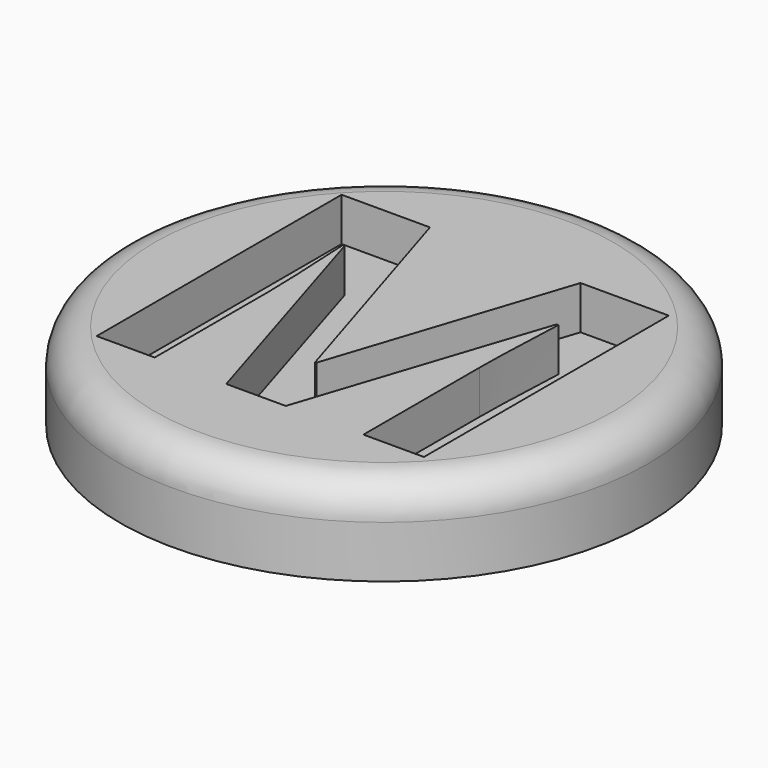
from build123d import *

# Parameters (mm, degrees)
F0_R         = 9.6561392052
F1_DEPTH     = 3.175
F2_R         = 1.27
F3_TEXT_SIZE = 15.6879974788
F4_DEPTH     = 1.5875


# Not quite as in the source:
# - Text() gives the source's letters only with a copy of the font that has no kerning and outlines rounded to 1/6400 em; it was checked with that copy


with BuildPart() as f1:
    # F0 (on Top) → F1 (new body)
    with BuildSketch(Plane.XY):
        Circle(F0_R)
    extrude(amount=F1_DEPTH)

    # F2
    f2_edges = [f1.edges().sort_by_distance(p)[0] for p in [
        (-9.656139, 0, 3.175),
    ]]
    fillet(f2_edges, radius=F2_R)

    # F3 (on face) → F4 (cut)
    with BuildSketch(Plane.XY.offset(3.175)):
        with Locations((-7.4662480183, -5.5725686252)):
            Text('M', F3_TEXT_SIZE, font='Open Sans', font_style=FontStyle.BOLD, text_align=(TextAlign.LEFT, TextAlign.BOTTOM))
    extrude(amount=-F4_DEPTH, mode=Mode.SUBTRACT)


solid = f1.part
